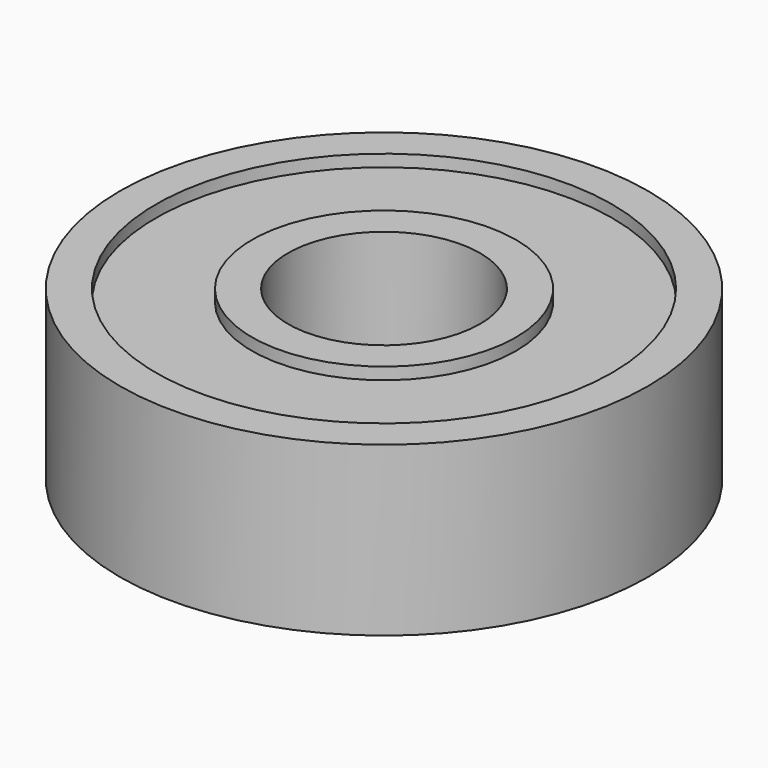
from build123d import *

# Parameters (mm, degrees)
F0_R     = 11
F0_R_2   = 9.5
F1_DEPTH = 3.5
F0_R_3   = 5.5
F0_R_4   = 4
F2_DEPTH = 3


with BuildPart() as f1:
    # F0 (on Top) → F1 (new body, symmetric)
    with BuildSketch(Plane.XY):
        Circle(F0_R)
        Circle(F0_R_2, mode=Mode.SUBTRACT)
    extrude(amount=F1_DEPTH, both=True)



with BuildPart() as f1b:
    # F0 (on Top) → F1, piece 2 (new body, symmetric)
    with BuildSketch(Plane.XY):
        Circle(F0_R_3)
        Circle(F0_R_4, mode=Mode.SUBTRACT)
    extrude(amount=F1_DEPTH, both=True)


with BuildPart() as f1_1:
    add(f1.part)

    add(f1b.part)  # F2 merges F1b
    # F0 (on Top) → F2 (join, symmetric)
    with BuildSketch(Plane.XY):
        Circle(F0_R_2)
        Circle(F0_R_3, mode=Mode.SUBTRACT)
    extrude(amount=F2_DEPTH, both=True)


solid = f1_1.part
